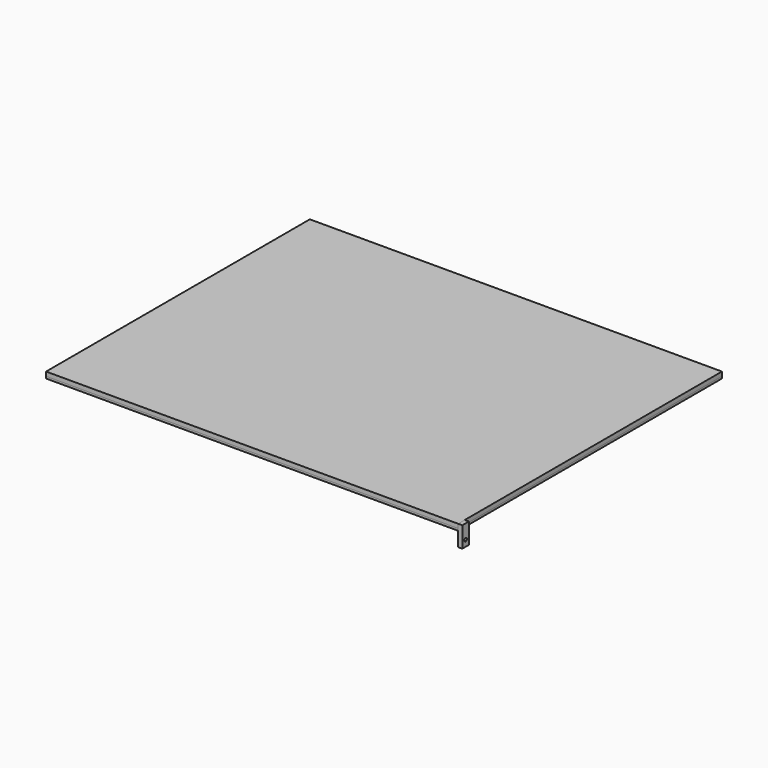
from build123d import *

# Parameters (mm, degrees)
F0_W     = 840
F0_H     = 80
F0_H_2   = 640
F1_DEPTH = 10
F2_DEPTH = 5
F3_W     = 20
F3_H     = 50
F3_R     = 4
F4_DEPTH = 10


# Not quite as in the source:
# - a feature names something its author has since deleted; it is built from what else it names


with BuildPart() as f1:
    # F0 (on Top) → F1 (new body)
    with BuildSketch(Plane.XY):
        Polygon((-446.064549312, 490.2843640471), (-446.064549312, -309.7156359529), (-366.064549312, -309.7156359529), (-366.064549312, -229.7156359529), (-366.064549312, 410.2843640471), (-366.064549312, 490.2843640471), align=None)
        with Locations((53.935450688, -269.7156359529)):
            Rectangle(F0_W, F0_H)
        Polygon((473.935450688, -229.7156359529), (473.935450688, -309.7156359529), (553.935450688, -309.7156359529), (553.935450688, 490.2843640471), (473.935450688, 490.2843640471), (473.935450688, 410.2843640471), align=None)
        with Locations((53.935450688, 90.2843640471)):
            Rectangle(F0_W, F0_H_2)
        with Locations((53.935450688, 450.2843640471)):
            Rectangle(F0_W, F0_H)
    extrude(amount=F1_DEPTH)


with BuildPart() as f2:
    # F0 (on Top) → F2 (new body)
    with BuildSketch(Plane.XY):
        Polygon((-446.064549312, 490.2843640471), (-446.064549312, -309.7156359529), (-366.064549312, -309.7156359529), (-366.064549312, -229.7156359529), (-366.064549312, 410.2843640471), (-366.064549312, 490.2843640471), align=None)
        with Locations((53.935450688, 450.2843640471)):
            Rectangle(F0_W, F0_H)
        with Locations((53.935450688, -269.7156359529)):
            Rectangle(F0_W, F0_H)
        Polygon((473.935450688, -229.7156359529), (473.935450688, -309.7156359529), (553.935450688, -309.7156359529), (553.935450688, 490.2843640471), (473.935450688, 490.2843640471), (473.935450688, 410.2843640471), align=None)
    extrude(amount=-F2_DEPTH)


with BuildPart() as f4:
    # F3 (on face) → F4 (new body)
    with BuildSketch(Plane.YZ.offset(553.935450688)):
        with Locations((-299.7156359529, -15)):
            Rectangle(F3_W, F3_H)
        with Locations((-299.7156359529, -25)):
            Circle(F3_R, mode=Mode.SUBTRACT)
    extrude(amount=F4_DEPTH)


solid = Compound([f1.part, f2.part, f4.part])
